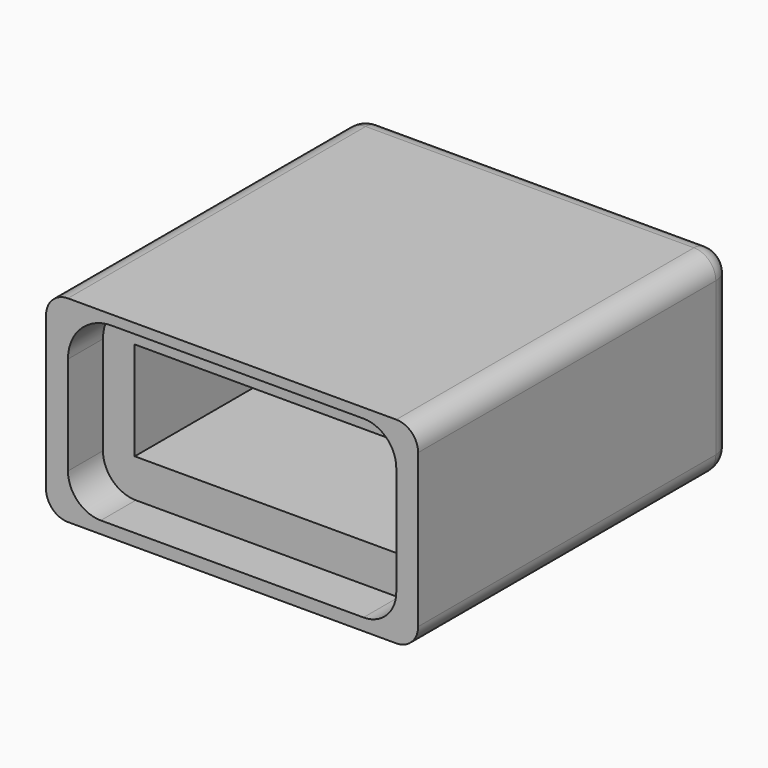
from build123d import *

# Parameters (mm, degrees)
F1_DEPTH = 18
F2_W     = 12.1
F2_H     = 4.5
F3_DEPTH = 14.43852
F5_DEPTH = 2
F6_R     = 1


# Not quite as in the source:
# - a feature names something its author has since deleted; it is built from what else it names


with BuildPart() as f1:
    # F0 (on Front) → F1 (new body)
    with BuildSketch(Plane.XZ):
        with BuildLine():
            ThreePointArc((8.5, 3.4460804202), (8.2071067812, 4.1531872014), (7.5, 4.4460804202))
            Line((7.5, 4.4460804202), (-7.5, 4.4460804202))
            ThreePointArc((-7.5, 4.4460804202), (-8.2071067812, 4.1531872014), (-8.5, 3.4460804202))
            Line((-8.5, 3.4460804202), (-8.5, -3.5539195798))
            ThreePointArc((-8.5, -3.5539195798), (-8.2071067812, -4.261026361), (-7.5, -4.5539195798))
            Line((-7.5, -4.5539195798), (7.5, -4.5539195798))
            ThreePointArc((7.5, -4.5539195798), (8.2071067812, -4.261026361), (8.5, -3.5539195798))
            Line((8.5, -3.5539195798), (8.5, 3.4460804202))
        make_face()
    extrude(amount=-F1_DEPTH)

    # F2 (on face) → F3 (cut)
    with BuildSketch(Plane.XZ):
        Rectangle(F2_W, F2_H)
    extrude(amount=-F3_DEPTH, mode=Mode.SUBTRACT)

    # F4 (on face) → F5 (cut)
    with BuildSketch(Plane.XZ):
        with BuildLine():
            Line((-6, -4), (6, -4))
            ThreePointArc((6, -4), (7.0606601718, -3.5606601718), (7.5, -2.5))
            Line((7.5, -2.5), (7.5, 2.5))
            ThreePointArc((7.5, 2.5), (7.0606601718, 3.5606601718), (6, 4))
            Line((6, 4), (-5.5, 4))
            ThreePointArc((-5.5, 4), (-6.9142135624, 3.4142135624), (-7.5, 2))
            Line((-7.5, 2), (-7.5, -2.5))
            ThreePointArc((-7.5, -2.5), (-7.0606601718, -3.5606601718), (-6, -4))
        make_face()
    extrude(amount=-F5_DEPTH, mode=Mode.SUBTRACT)

    # F6
    f6_edges = [f1.edges().sort_by_distance(p)[0] for p in [
        (8.207107, 18, -4.261026),
        (8.5, 18, -0.05392),
        (8.207107, 18, 4.153187),
        (0, 18, 4.44608),
        (-8.207107, 18, 4.153187),
        (-8.5, 18, -0.05392),
        (-8.207107, 18, -4.261026),
        (0, 18, -4.55392),
    ]]
    fillet(f6_edges, radius=F6_R)


solid = f1.part
